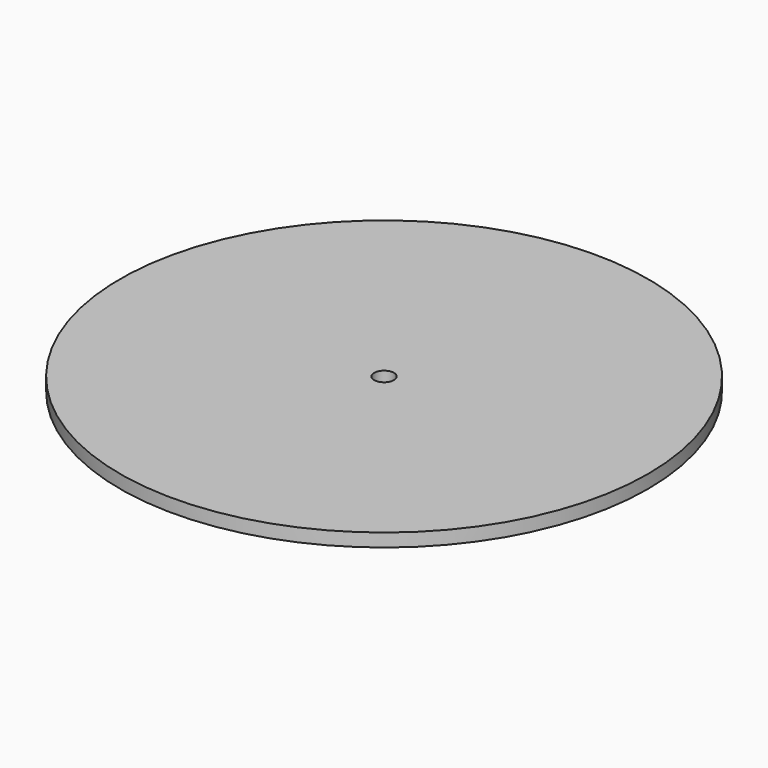
from build123d import *

# Parameters (mm, degrees)
F0_R     = 63.5
F0_R_2   = 2.38125
F1_DEPTH = 3.175


# Not quite as in the source:
# - a length typed as a fraction of an inch, garbled in the dataset ("3 / 203.2 mm" for 3/8 in), is restored


with BuildPart() as f1:
    # F0 (on Top) → F1 (new body)
    with BuildSketch(Plane.XY):
        Circle(F0_R)
        Circle(F0_R_2, mode=Mode.SUBTRACT)
    extrude(amount=F1_DEPTH)


solid = f1.part
